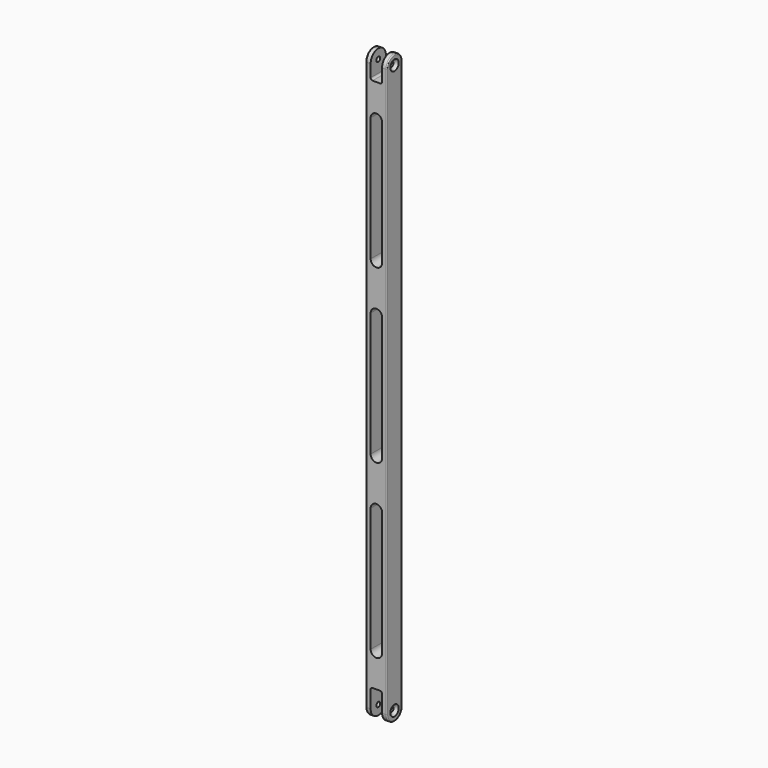
from build123d import *

# Parameters (mm, degrees)
F0_W      = 22
F0_H      = 615
F1_DEPTH  = 20
F2_W      = 12
F2_H      = 20
F3_DEPTH  = 25
F4_W      = 12
F4_H      = 20
F5_DEPTH  = 30
F6_R      = 9.99999
F7_R      = 2.5
F8_DEPTH  = 30
F10_DEPTH = 25
F11_R     = 1
F12_SIZE  = 3
F13_R     = 2


# Not quite as in the source:
# - a fillet or chamfer is up to 0.001 mm smaller than in the source, because OpenCascade refuses the exact size


with BuildPart() as f1:
    # F0 (on Front) → F1 (new body)
    with BuildSketch(Plane.XZ):
        Rectangle(F0_W, F0_H)
    extrude(amount=F1_DEPTH)

    # F2 (on face) → F3 (cut)
    with BuildSketch(Plane.XY.offset(307.5)):
        with Locations((0, -10)):
            Rectangle(F2_W, F2_H)
    extrude(amount=-F3_DEPTH, mode=Mode.SUBTRACT)

    # F4 (on face) → F5 (cut)
    with BuildSketch(Plane(origin=(0, 0, -307.5), x_dir=(1, 0, 0), z_dir=(0, 0, -1))):
        with Locations((0, 10)):
            Rectangle(F4_W, F4_H)
    extrude(amount=-F5_DEPTH, mode=Mode.SUBTRACT)

    # F6 (radius 10 in the source; OpenCascade refuses exactly that, so slightly less here)
    f6_edges = [f1.edges().sort_by_distance(p)[0] for p in [
        (-8.5, 0, -307.5),
        (8.5, 0, -307.5),
        (8.5, -20, -307.5),
        (-8.5, -20, -307.5),
        (-8.5, -20, 307.5),
        (-8.5, 0, 307.5),
        (8.5, 0, 307.5),
        (8.5, -20, 307.5),
    ]]
    fillet(f6_edges, radius=F6_R)

    # F7 (on face) → F8 (cut)
    with BuildSketch(Plane(origin=(-11, 0, 0), x_dir=(0, -1, 0), z_dir=(-1, 0, 0))):
        with Locations((10, 297.5)):
            Circle(F7_R)
        with Locations((10, -297.5)):
            Circle(F7_R)
    extrude(amount=-F8_DEPTH, mode=Mode.SUBTRACT)

    # F9 (on face) → F10 (cut)
    with BuildSketch(Plane.XZ.offset(20)):
        with BuildLine():
            ThreePointArc((6, 247.5), (0, 253.5), (-6, 247.5))
            Line((-6, 247.5), (-6, 117.5))
            ThreePointArc((-6, 117.5), (0, 111.5), (6, 117.5))
            Line((6, 117.5), (6, 247.5))
        make_face()
        with BuildLine():
            ThreePointArc((-6, -62.5), (0, -68.5), (6, -62.5))
            Line((6, -62.5), (6, 67.5))
            ThreePointArc((6, 67.5), (0, 73.5), (-6, 67.5))
            Line((-6, 67.5), (-6, -62.5))
        make_face()
        with BuildLine():
            Line((-6, -112.5), (-6, -242.5))
            ThreePointArc((-6, -242.5), (0, -248.5), (6, -242.5))
            Line((6, -242.5), (6, -112.5))
            ThreePointArc((6, -112.5), (0, -106.5), (-6, -112.5))
        make_face()
    extrude(amount=-F10_DEPTH, mode=Mode.SUBTRACT)

    # F11
    f11_edges = [f1.edges().sort_by_distance(p)[0] for p in [
        (11, 0, 0),
        (-11, 0, 0),
    ]]
    fillet(f11_edges, radius=F11_R)

    # F12
    f12_edges = [f1.edges().sort_by_distance(p)[0] for p in [
        (11, -7.5, 297.5),
        (11, -7.5, -297.5),
    ]]
    chamfer(f12_edges, length=F12_SIZE)

    # F13
    f13_edges = [f1.edges().sort_by_distance(p)[0] for p in [
        (-6, -10, -277.5),
        (6, -10, -277.5),
        (6, -10, 282.5),
        (-6, -10, 282.5),
    ]]
    fillet(f13_edges, radius=F13_R)


solid = f1.part
